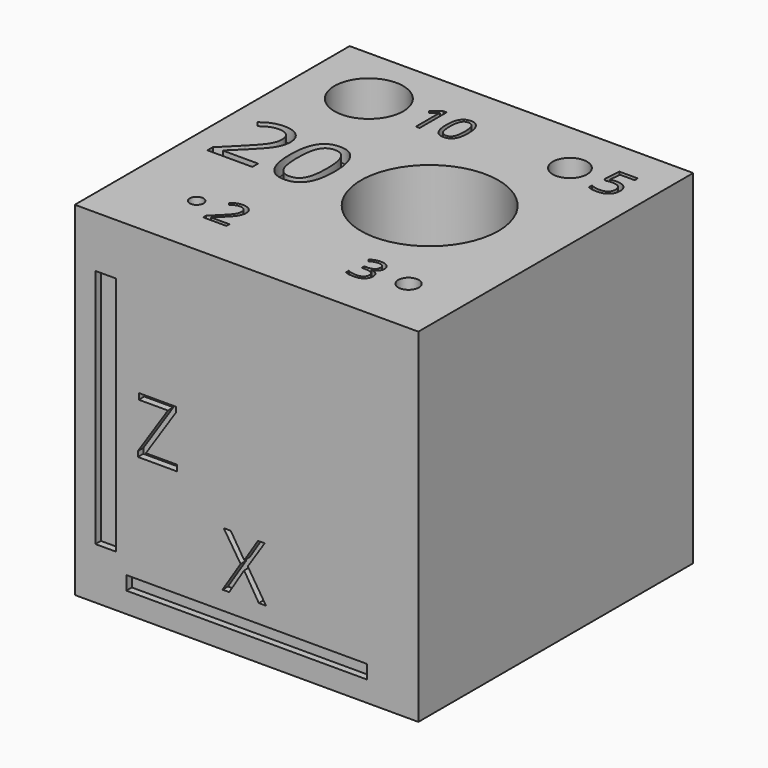
from build123d import *

# Parameters (mm, degrees)
F0_W           = 50
F0_H           = 50
F1_DEPTH       = 50
F2_W           = 35
F2_H           = 2
F2_W_2         = 3
F2_H_2         = 35
F2_TEXT_SIZE   = 11.536619824
F2_TEXT_SIZE_2 = 11.1261601716
F4_DEPTH       = 1
F3_TEXT_SIZE   = 10.1803589661
F3_W           = 35
F3_H           = 3
F5_DEPTH       = 1
F6_R           = 5
F6_R_2         = 10
F6_R_3         = 2.5
F6_R_4         = 1.5
F6_R_5         = 1
F7_DEPTH       = 50
F6_TEXT_SIZE   = 6.8933832356
F6_TEXT_SIZE_2 = 7.5061268742
F6_TEXT_SIZE_3 = 7.1997547315
F6_TEXT_SIZE_4 = 6.5104156319
F6_TEXT_SIZE_5 = 13.9399518957
F8_DEPTH       = 2


# Not quite as in the source:
# - Text() gives the source's letters only with a copy of the font that has no kerning and outlines rounded to 1/6400 em; it was checked with that copy


with BuildPart() as f1:
    # F0 (on Top) → F1 (new body)
    with BuildSketch(Plane.XY):
        Rectangle(F0_W, F0_H)
    extrude(amount=F1_DEPTH)

    # F2 (on face) → F4 (cut)
    with BuildSketch(Plane.XZ.offset(25)):
        with Locations((0, 4)):
            Rectangle(F2_W, F2_H)
        with Locations((-20.5, 25)):
            Rectangle(F2_W_2, F2_H_2)
        with Locations((-16.2814031485, 20.6711094146)):
            Text('Z', F2_TEXT_SIZE, font='Open Sans', text_align=(TextAlign.LEFT, TextAlign.BOTTOM))
        with Locations((-3.5499404798, 7.6734586024)):
            Text('X', F2_TEXT_SIZE_2, font='Open Sans', text_align=(TextAlign.LEFT, TextAlign.BOTTOM))
    extrude(amount=-F4_DEPTH, mode=Mode.SUBTRACT)

    # F3 (on face) → F5 (cut)
    with BuildSketch(Plane(origin=(-25, 0, 0), x_dir=(0, -1, 0), z_dir=(-1, 0, 0))):
        with Locations((-3.1805668364, 7.8468960437)):
            Text('Y', F3_TEXT_SIZE, font='Open Sans', text_align=(TextAlign.LEFT, TextAlign.BOTTOM))
        with Locations((0, 4.5)):
            Rectangle(F3_W, F3_H)
    extrude(amount=-F5_DEPTH, mode=Mode.SUBTRACT)

    # F6 (on face) → F7 (cut, through all)
    with BuildSketch(Plane.XY.offset(50)):
        with Locations((-15.2205890045, 16.2683818489)):
            Circle(F6_R)
        with Locations((6.6268551132, 0.0251705185)):
            Circle(F6_R_2)
        with Locations((13.290441595, 17.2058828175)):
            Circle(F6_R_3)
        with Locations((16.7647060007, -16.4889711887)):
            Circle(F6_R_4)
        with Locations((-14.779413119, -15.6066184863)):
            Circle(F6_R_5)
    extrude(amount=-F7_DEPTH, mode=Mode.SUBTRACT)

    # F6 (on face) → F8 (cut)
    with BuildSketch(Plane.XY.offset(50)):
        with Locations((6.6268551132, 0.0251705185)):
            Circle(F6_R_2)
        with Locations((-15.2205890045, 16.2683818489)):
            Circle(F6_R)
        with Locations((13.290441595, 17.2058828175)):
            Circle(F6_R_3)
        with Locations((16.7647060007, -16.4889711887)):
            Circle(F6_R_4)
        with Locations((-14.779413119, -15.6066184863)):
            Circle(F6_R_5)
        with Locations((-8.6029421, 14.2279416323)):
            Text('10', F6_TEXT_SIZE, font='Open Sans', text_align=(TextAlign.LEFT, TextAlign.BOTTOM))
        with Locations((17.4264749512, 14.6691170521)):
            Text('5', F6_TEXT_SIZE_2, font='Open Sans', text_align=(TextAlign.LEFT, TextAlign.BOTTOM))
        with Locations((-12.0220580138, -18.3088239282)):
            Text('2', F6_TEXT_SIZE_3, font='Open Sans', text_align=(TextAlign.LEFT, TextAlign.BOTTOM))
        with Locations((9.1544110328, -18.9154408872)):
            Text('3', F6_TEXT_SIZE_4, font='Open Sans', text_align=(TextAlign.LEFT, TextAlign.BOTTOM))
        with Locations((-22.279413417, -5.1286768576)):
            Text('20', F6_TEXT_SIZE_5, font='Open Sans', text_align=(TextAlign.LEFT, TextAlign.BOTTOM))
    extrude(amount=-F8_DEPTH, mode=Mode.SUBTRACT)


solid = f1.part
